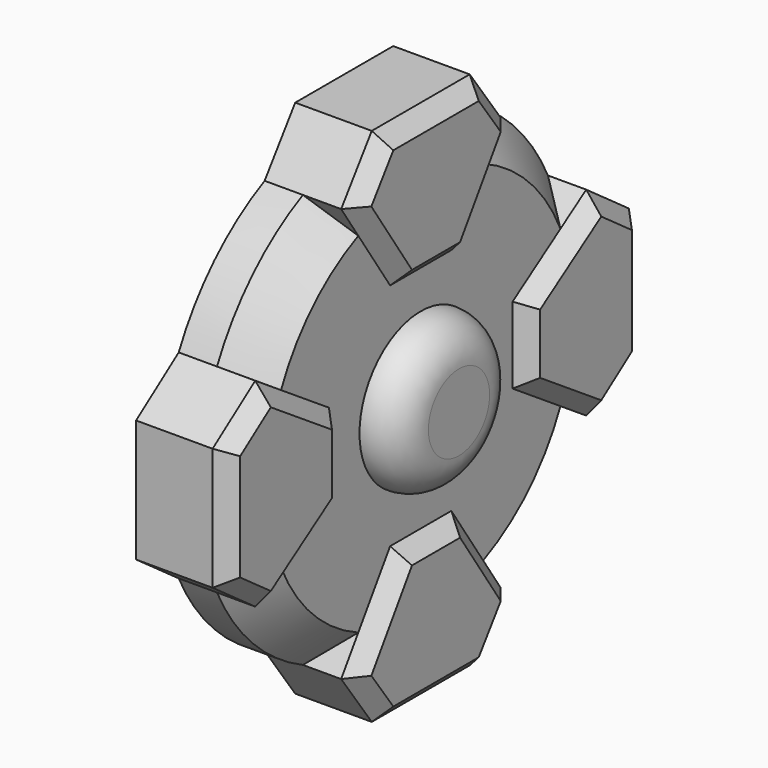
from build123d import *

# Parameters (mm, degrees)
F1_DEPTH = 10
F2_DEPTH = 12
F3_SIZE  = 5
F4_SIZE  = 1.99999
F5_R     = 10
F6_DEPTH = 5
F7_R     = 4.99999
F9_DEPTH = 3


# Not quite as in the source:
# - a fillet or chamfer is up to 0.001 mm smaller than in the source, because OpenCascade refuses the exact size


with BuildPart() as f1:
    # F0 (on Right) → F1 (new body)
    with BuildSketch(Plane.YZ):
        with BuildLine():
            Line((15, 5), (27.0370116692, 13))
            ThreePointArc((27.0370116692, 13), (21.2132034356, 21.2132034356), (13, 27.0370116692))
            Line((13, 27.0370116692), (5, 15))
            Line((5, 15), (0, 15))
            Line((0, 15), (-5, 15))
            Line((-5, 15), (-13, 27.0370116692))
            ThreePointArc((-13, 27.0370116692), (-21.2132034356, 21.2132034356), (-27.0370116692, 13))
            Line((-27.0370116692, 13), (-15, 5))
            Line((-15, 5), (-15, 0))
            Line((-15, 0), (-15, -5))
            Line((-15, -5), (-27.0370116692, -13))
            ThreePointArc((-27.0370116692, -13), (-21.2132034356, -21.2132034356), (-13, -27.0370116692))
            Line((-13, -27.0370116692), (-5, -15))
            Line((-5, -15), (0, -15))
            Line((0, -15), (5, -15))
            Line((5, -15), (13, -27.0370116692))
            ThreePointArc((13, -27.0370116692), (21.2132034356, -21.2132034356), (27.0370116692, -13))
            Line((27.0370116692, -13), (15, -5))
            Line((15, -5), (15, 0))
            Line((15, 0), (15, 5))
        make_face()
    extrude(amount=F1_DEPTH)

    # F0 (on Right) → F2 (join)
    with BuildSketch(Plane.YZ):
        with BuildLine():
            ThreePointArc((27.0370116692, -13), (29.2498747867, -6.6666952054), (30, 0))
            ThreePointArc((30, 0), (29.2498747867, 6.6666952054), (27.0370116692, 13))
            Line((27.0370116692, 13), (15, 5))
            Line((15, 5), (15, 0))
            Line((15, 0), (15, -5))
            Line((15, -5), (27.0370116692, -13))
        make_face()
        with BuildLine():
            ThreePointArc((27.0370116692, 13), (29.2498747867, 6.6666952054), (30, 0))
            ThreePointArc((30, 0), (29.2498747867, -6.6666952054), (27.0370116692, -13))
            Line((27.0370116692, -13), (34, -8))
            Line((34, -8), (34, 0))
            Line((34, 0), (34, 8))
            Line((34, 8), (27.0370116692, 13))
        make_face()
        with BuildLine():
            Line((5, 15), (13, 27.0370116692))
            ThreePointArc((13, 27.0370116692), (0, 30), (-13, 27.0370116692))
            Line((-13, 27.0370116692), (-5, 15))
            Line((-5, 15), (0, 15))
            Line((0, 15), (5, 15))
        make_face()
        with BuildLine():
            ThreePointArc((-13, 27.0370116692), (0, 30), (13, 27.0370116692))
            Line((13, 27.0370116692), (8, 34))
            Line((8, 34), (0, 34))
            Line((0, 34), (-8, 34))
            Line((-8, 34), (-13, 27.0370116692))
        make_face()
        with BuildLine():
            Line((-15, 5), (-27.0370116692, 13))
            ThreePointArc((-27.0370116692, 13), (-30, 0), (-27.0370116692, -13))
            Line((-27.0370116692, -13), (-15, -5))
            Line((-15, -5), (-15, 0))
            Line((-15, 0), (-15, 5))
        make_face()
        with BuildLine():
            ThreePointArc((-27.0370116692, -13), (-30, 0), (-27.0370116692, 13))
            Line((-27.0370116692, 13), (-34, 8))
            Line((-34, 8), (-34, 0))
            Line((-34, 0), (-34, -8))
            Line((-34, -8), (-27.0370116692, -13))
        make_face()
        with BuildLine():
            ThreePointArc((-13, -27.0370116692), (0, -30), (13, -27.0370116692))
            Line((13, -27.0370116692), (5, -15))
            Line((5, -15), (0, -15))
            Line((0, -15), (-5, -15))
            Line((-5, -15), (-13, -27.0370116692))
        make_face()
        with BuildLine():
            Line((8, -34), (13, -27.0370116692))
            ThreePointArc((13, -27.0370116692), (0, -30), (-13, -27.0370116692))
            Line((-13, -27.0370116692), (-8, -34))
            Line((-8, -34), (0, -34))
            Line((0, -34), (8, -34))
        make_face()
    extrude(amount=F2_DEPTH)

    # F3
    f3_edges = [f1.edges().sort_by_distance(p)[0] for p in [
        (10, 21.213203, 21.213203),
        (10, -21.213203, 21.213203),
        (10, -21.213203, -21.213203),
        (10, 21.213203, -21.213203),
    ]]
    chamfer(f3_edges, length=F3_SIZE)

    # F4 (size 2 in the source; OpenCascade refuses exactly that, so slightly less here)
    f4_edges = [f1.edges().sort_by_distance(p)[0] for p in [
        (12, 0, 34),
        (12, -10.5, 30.518506),
        (12, 10.5, 30.518506),
        (12, -9, 21.018506),
        (12, 9, 21.018506),
        (12, 0, 15),
        (12, -15, 0),
        (12, -21.018506, 9),
        (12, -30.518506, 10.5),
        (12, -34, 0),
        (12, -30.518506, -10.5),
        (12, -21.018506, -9),
        (12, 0, -15),
        (12, -9, -21.018506),
        (12, -10.5, -30.518506),
        (12, 0, -34),
        (12, 10.5, -30.518506),
        (12, 9, -21.018506),
        (12, 15, 0),
        (12, 21.018506, 9),
        (12, 30.518506, 10.5),
        (12, 34, 0),
        (12, 21.018506, -9),
        (12, 30.518506, -10.5),
    ]]
    chamfer(f4_edges, length=F4_SIZE)

    # F5 (on face) → F6 (join)
    with BuildSketch(Plane.YZ.offset(10)):
        Circle(F5_R)
    extrude(amount=F6_DEPTH)

    # F7 (radius 5 in the source; OpenCascade refuses exactly that, so slightly less here)
    f7_edges = [f1.edges().sort_by_distance(p)[0] for p in [
        (15, -10, 0),
    ]]
    fillet(f7_edges, radius=F7_R)

    # F8 (on face) → F9 (cut)
    with BuildSketch(Plane.YZ):
        with BuildLine():
            ThreePointArc((0, -15), (10.6066017178, -10.6066017178), (15, 0))
            ThreePointArc((15, 0), (10.6066017178, 10.6066017178), (0, 15))
            ThreePointArc((0, 15), (-10.6066017178, 10.6066017178), (-15, 0))
            ThreePointArc((-15, 0), (-10.6066017178, -10.6066017178), (0, -15))
        make_face()
    extrude(amount=F9_DEPTH, mode=Mode.SUBTRACT)


solid = f1.part
